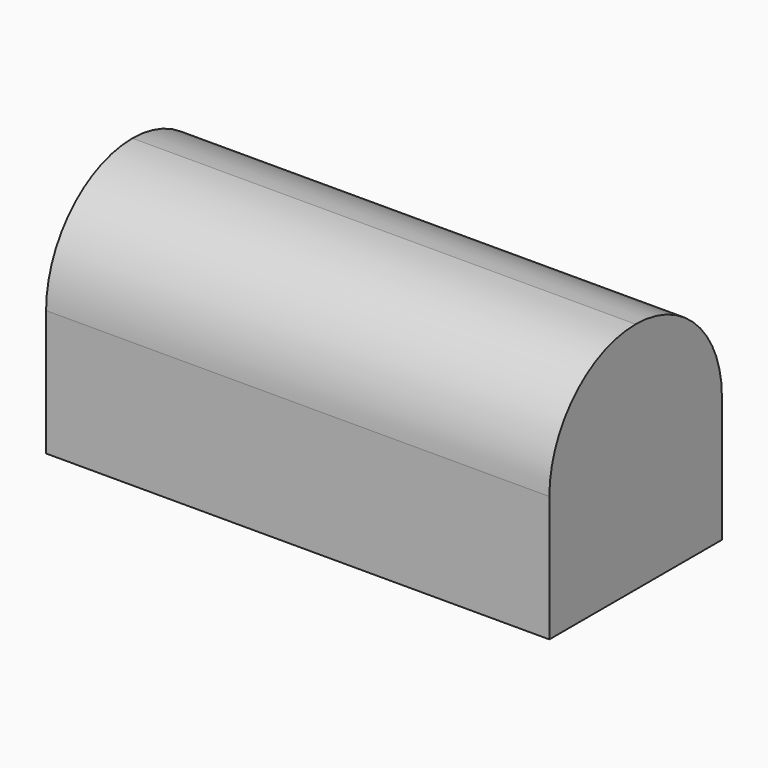
from build123d import *

# Parameters (mm, degrees)
F0_W     = 7
F0_H     = 3
F1_DEPTH = 3.25
F2_R     = 1.49999


# Not quite as in the source:
# - a fillet or chamfer is up to 0.001 mm smaller than in the source, because OpenCascade refuses the exact size


with BuildPart() as f1:
    # F0 (on Top) → F1 (new body)
    with BuildSketch(Plane.XY):
        Rectangle(F0_W, F0_H)
    extrude(amount=F1_DEPTH)

    # F2 (radius 1.5 in the source; OpenCascade refuses exactly that, so slightly less here)
    f2_edges = [f1.edges().sort_by_distance(p)[0] for p in [
        (0, -1.5, 3.25),
        (0, 1.5, 3.25),
    ]]
    fillet(f2_edges, radius=F2_R)


solid = f1.part
